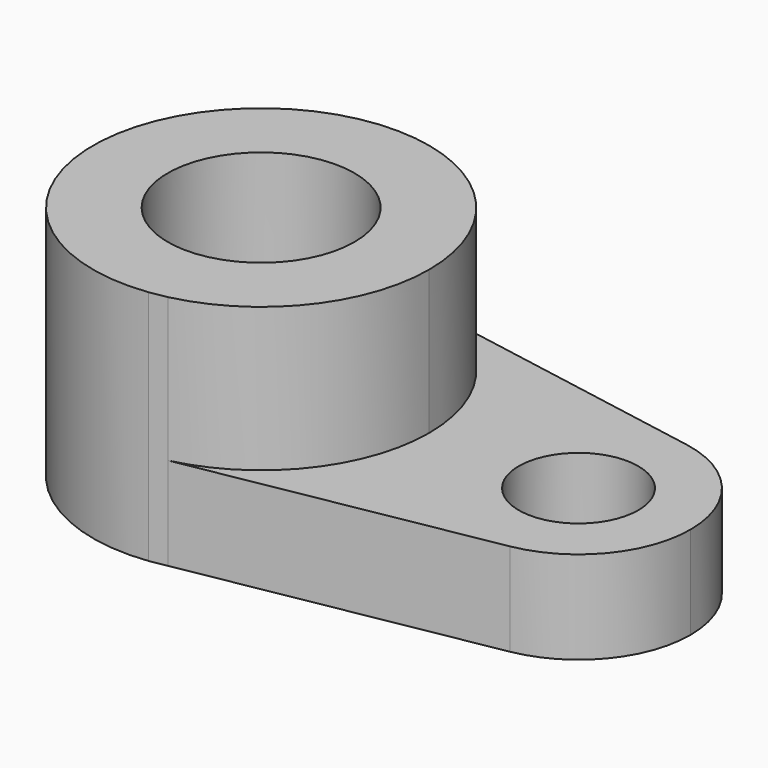
from build123d import *

# Parameters (mm, degrees)
F0_R     = 15.875
F0_R_2   = 10.16
F1_DEPTH = 15.7734
F2_R     = 15.875
F3_DEPTH = 24.4602


with BuildPart() as f1:
    # F0 (on Top) → F1 (new body)
    with BuildSketch(Plane.XY):
        with BuildLine():
            Line((6.4681247744, 27.833325114), (3.5634199556, 28.3519428474))
            ThreePointArc((3.5634199556, 28.3519428474), (-28.575, 0), (3.5634199556, -28.3519428474))
            Line((3.5634199556, -28.3519428474), (6.4681247744, -27.833325114))
            ThreePointArc((6.4681247744, -27.833325114), (22.3758495976, -17.7722249532), (28.575, 0))
            ThreePointArc((28.575, 0), (22.3758495976, 17.7722249532), (6.4681247744, 27.833325114))
        make_face()
        Circle(F0_R, mode=Mode.SUBTRACT)
        with BuildLine():
            Line((57.3233139044, 18.7534341921), (6.4681247744, 27.833325114))
            ThreePointArc((6.4681247744, 27.833325114), (22.3758495976, 17.7722249532), (28.575, 0))
            ThreePointArc((28.575, 0), (22.3758495976, -17.7722249532), (6.4681247744, -27.833325114))
            Line((6.4681247744, -27.833325114), (57.3233139044, -18.7534341921))
            ThreePointArc((57.3233139044, -18.7534341921), (34.925, 0), (57.3233139044, 18.7534341921))
        make_face()
        with BuildLine():
            ThreePointArc((73.025, 0), (68.5812979546, 12.2294137251), (57.3233139044, 18.7534341921))
            ThreePointArc((57.3233139044, 18.7534341921), (34.925, 0), (57.3233139044, -18.7534341921))
            ThreePointArc((57.3233139044, -18.7534341921), (68.5812979546, -12.2294137251), (73.025, 0))
        make_face()
        with Locations((53.975, 0)):
            Circle(F0_R_2, mode=Mode.SUBTRACT)
    extrude(amount=F1_DEPTH)

    # F2 (on face) → F3 (join)
    with BuildSketch(Plane.XY.offset(15.7734)):
        with BuildLine():
            Line((6.4681247744, 27.833325114), (3.5634199556, 28.3519428474))
            ThreePointArc((3.5634199556, 28.3519428474), (-28.575, 0), (3.5634199556, -28.3519428474))
            Line((3.5634199556, -28.3519428474), (6.4681247744, -27.833325114))
            ThreePointArc((6.4681247744, -27.833325114), (22.3758495976, -17.7722249532), (28.575, 0))
            ThreePointArc((28.575, 0), (22.3758495976, 17.7722249532), (6.4681247744, 27.833325114))
        make_face()
        Circle(F2_R, mode=Mode.SUBTRACT)
    extrude(amount=F3_DEPTH)


solid = f1.part
